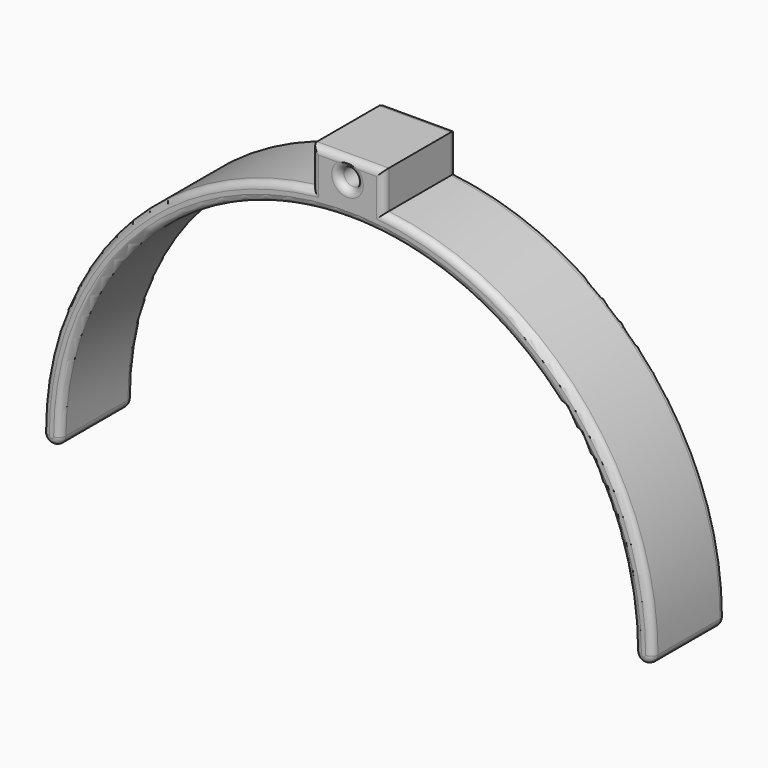
from build123d import *

# Parameters (mm, degrees)
F0_R         = 2.5
F1_DEPTH     = 25.4
F2_T1_DEPTH  = 29.525
F2_T4_ANGLE  = 180
F2_T6_ANGLE  = 180
F2_T8_ANGLE  = 180
F2_T12_ANGLE = 86.4550249792
F2_T17_DEPTH = 20.1152849193
F2_S18_R     = 85
F2_T19_DEPTH = 12
F2_T23_DEPTH = 20.1152849193
F2_S24_R     = 85
F2_T25_DEPTH = 12
F2_T29_ANGLE = 86.4550249792
F2_T37_ANGLE = 86.4550249792
F2_T41_DEPTH = 20.1152849193
F2_S42_R     = 85
F2_T43_DEPTH = 12
F2_T49_DEPTH = 20.1152849193
F2_S50_R     = 85
F2_T51_DEPTH = 12
F2_T54_ANGLE = 86.4550249792
F3_T3_ANGLE  = 180
F3_T6_ANGLE  = 180
F3_T9_ANGLE  = 180
F3_T12_ANGLE = 86.4550249792
F3_T16_DEPTH = 20.1152849193
F3_S17_R     = 85
F3_T18_DEPTH = 12
F3_T21_DEPTH = 29.525
F3_T24_DEPTH = 20.1152849193
F3_S25_R     = 85
F3_T26_DEPTH = 12
F3_T29_ANGLE = 86.4550249792
F3_T37_DEPTH = 20.1152849193
F3_S38_R     = 85
F3_T39_DEPTH = 12
F3_T42_ANGLE = 86.4550249792
F3_T48_ANGLE = 86.4550249792
F3_T52_DEPTH = 20.1152849193
F3_S53_R     = 85
F3_T54_DEPTH = 12


# Not quite as in the source:
# - a fillet or chamfer that OpenCascade refuses, or shapes differently, is made with other operations: its cross-section is extruded or revolved along the edge and cut away or added


with BuildPart() as f1:
    # F0 (on Front) → F1 (new body)
    with BuildSketch(Plane.XZ):
        with BuildLine():
            ThreePointArc((-80, 0), (0, 80), (80, 0))
            ThreePointArc((80, 0), (82.5, -2.5), (85, 0))
            ThreePointArc((85, 0), (63.5413251357, 56.4579489532), (10, 84.4097150807))
            Line((10, 84.4097150807), (10, 95))
            Line((10, 95), (0, 95))
            Line((0, 95), (-10, 95))
            Line((-10, 95), (-10, 84.4097150807))
            ThreePointArc((-10, 84.4097150807), (-63.5413251357, 56.4579489532), (-85, 0))
            ThreePointArc((-85, 0), (-82.5, -2.5), (-80, 0))
        make_face()
        with Locations((0, 89.7048575403)):
            Circle(F0_R, mode=Mode.SUBTRACT)
    extrude(amount=F1_DEPTH)

    # F2: fillet of radius 1.905 on 9 edges, made by hand

    # F2_s2 → F2_t1 (cut)
    with BuildSketch(Plane.YZ.offset(-14.7625)):
        with BuildLine():
            ThreePointArc((-25.4, 93.095), (-24.8420384182, 94.4420384182), (-23.495, 95))
            Line((-23.495, 95), (-25.4, 95))
            Line((-25.4, 95), (-25.4, 93.095))
        make_face()
    extrude(amount=F2_T1_DEPTH, mode=Mode.SUBTRACT)

    # F2_s3 → F2_t4 (revolve, cut)
    with BuildSketch(Plane.XY):
        with BuildLine():
            ThreePointArc((-85, -23.495), (-84.4420384182, -24.8420384182), (-83.095, -25.4))
            Line((-83.095, -25.4), (-85, -25.4))
            Line((-85, -25.4), (-85, -23.495))
        make_face()
    revolve(axis=Axis((-82.5, -25.4, 0), (0, -1, 0)), revolution_arc=F2_T4_ANGLE, mode=Mode.SUBTRACT)

    # F2_s5 → F2_t6 (revolve, cut)
    with BuildSketch(Plane.XY):
        with BuildLine():
            ThreePointArc((-81.905, -25.4), (-80.5579615818, -24.8420384182), (-80, -23.495))
            Line((-80, -23.495), (-80, -25.4))
            Line((-80, -25.4), (-81.905, -25.4))
        make_face()
    revolve(axis=Axis((0, -25.4, 0), (0, 1, 0)), revolution_arc=F2_T6_ANGLE, mode=Mode.SUBTRACT)

    # F2_s7 → F2_t8 (revolve, cut)
    with BuildSketch(Plane.XY):
        with BuildLine():
            ThreePointArc((81.905, -25.4), (80.5579615818, -24.8420384182), (80, -23.495))
            Line((80, -23.495), (80, -25.4))
            Line((80, -25.4), (81.905, -25.4))
        make_face()
    revolve(axis=Axis((82.5, -25.4, 0), (0, -1, 0)), revolution_arc=F2_T8_ANGLE, mode=Mode.SUBTRACT)


with BuildPart() as f2_tool10:
    # F2_s11 → F2_t12 (revolve)
    with BuildSketch(Plane.XY):
        with BuildLine():
            ThreePointArc((83.095, -25.4), (84.4420384182, -24.8420384182), (85, -23.495))
            Line((85, -23.495), (85, -25.4))
            Line((85, -25.4), (83.095, -25.4))
        make_face()
    revolve(axis=Axis((0, -25.4, 0), (0, -1, 0)), revolution_arc=F2_T12_ANGLE)

    split(bisect_by=Plane.YZ.offset(10), keep=Keep.TOP)


with BuildPart() as f1_1:
    add(f1.part)

    # F2_t9: cut F2_tool10
    add(f2_tool10.part, mode=Mode.SUBTRACT)


with BuildPart() as f2_tool15:
    # F2_s16 → F2_t17 (new body)
    with BuildSketch(Plane.XY.offset(79.6472150807)):
        with BuildLine():
            ThreePointArc((8.095, -25.4), (9.4420384182, -24.8420384182), (10, -23.495))
            Line((10, -23.495), (10, -25.4))
            Line((10, -25.4), (8.095, -25.4))
        make_face()
    extrude(amount=F2_T17_DEPTH)

    # F2_s18 → F2_t19 (cut, symmetric)
    with BuildSketch(Plane.XZ.offset(24.4)):
        Circle(F2_S18_R)
    extrude(amount=F2_T19_DEPTH, both=True, mode=Mode.SUBTRACT)


with BuildPart() as f1_2:
    add(f1_1.part)

    # F2_t14: cut F2_tool15
    add(f2_tool15.part, mode=Mode.SUBTRACT)


with BuildPart() as f2_tool21:
    # F2_s22 → F2_t23 (new body)
    with BuildSketch(Plane.XY.offset(99.7625)):
        with BuildLine():
            ThreePointArc((-8.095, -25.4), (-9.4420384182, -24.8420384182), (-10, -23.495))
            Line((-10, -23.495), (-10, -25.4))
            Line((-10, -25.4), (-8.095, -25.4))
        make_face()
    extrude(amount=-F2_T23_DEPTH)

    # F2_s24 → F2_t25 (cut, symmetric)
    with BuildSketch(Plane.XZ.offset(24.4)):
        Circle(F2_S24_R)
    extrude(amount=F2_T25_DEPTH, both=True, mode=Mode.SUBTRACT)


with BuildPart() as f1_3:
    add(f1_2.part)

    # F2_t20: cut F2_tool21
    add(f2_tool21.part, mode=Mode.SUBTRACT)


with BuildPart() as f2_tool27:
    # F2_s28 → F2_t29 (revolve)
    with BuildSketch(Plane(origin=(0, 0, 0), x_dir=(0, 1, 0), z_dir=(0.9980865701, 0, 0.0618320187))):
        with BuildLine():
            ThreePointArc((-25.4, 83.095), (-24.8420384182, 84.4420384182), (-23.495, 85))
            Line((-23.495, 85), (-25.4, 85))
            Line((-25.4, 85), (-25.4, 83.095))
        make_face()
    revolve(axis=Axis((0, -25.4, 0), (0, -1, 0)), revolution_arc=F2_T29_ANGLE)

    split(bisect_by=Plane.YZ.offset(-10), keep=Keep.BOTTOM)


with BuildPart() as f1_4:
    add(f1_3.part)

    # F2_t26: cut F2_tool27
    add(f2_tool27.part, mode=Mode.SUBTRACT)

    # F2_s31 → F2_t32 (revolve, cut)
    with BuildSketch(Plane.XY.offset(89.7048575403)):
        with BuildLine():
            ThreePointArc((4.405, -25.4), (3.0579615818, -24.8420384182), (2.5, -23.495))
            Line((2.5, -23.495), (2.5, -25.4))
            Line((2.5, -25.4), (4.405, -25.4))
        make_face()
    revolve(axis=Axis((0, -25.4, 89.7048575403), (0, -1, 0)), mode=Mode.SUBTRACT)


with BuildPart() as f2_tool35:
    # F2_s36 → F2_t37 (revolve)
    with BuildSketch(Plane.XY):
        with BuildLine():
            ThreePointArc((83.095, -25.4), (84.4420384182, -24.8420384182), (85, -23.495))
            Line((85, -23.495), (85, -25.4))
            Line((85, -25.4), (83.095, -25.4))
        make_face()
    revolve(axis=Axis((0, -25.4, 0), (0, -1, 0)), revolution_arc=F2_T37_ANGLE)

    split(bisect_by=Plane.YZ.offset(10), keep=Keep.BOTTOM)


with BuildPart() as f2_tool39:
    # F2_s40 → F2_t41 (new body)
    with BuildSketch(Plane.XY.offset(79.6472150807)):
        with BuildLine():
            ThreePointArc((8.095, -25.4), (9.4420384182, -24.8420384182), (10, -23.495))
            Line((10, -23.495), (10, -25.4))
            Line((10, -25.4), (8.095, -25.4))
        make_face()
    extrude(amount=F2_T41_DEPTH)

    # F2_s42 → F2_t43 (intersect, symmetric)
    with BuildSketch(Plane.XZ.offset(24.4)):
        Circle(F2_S42_R)
    extrude(amount=F2_T43_DEPTH, both=True, mode=Mode.INTERSECT)


with BuildPart() as f2_tool35_1:
    add(f2_tool35.part)

    # F2_t44: intersect F2_tool39
    add(f2_tool39.part, mode=Mode.INTERSECT)


with BuildPart() as f1_5:
    add(f1_4.part)

    # F2_t33: cut F2_tool35
    add(f2_tool35_1.part, mode=Mode.SUBTRACT)


with BuildPart() as f2_tool47:
    # F2_s48 → F2_t49 (new body)
    with BuildSketch(Plane.XY.offset(99.7625)):
        with BuildLine():
            ThreePointArc((-8.095, -25.4), (-9.4420384182, -24.8420384182), (-10, -23.495))
            Line((-10, -23.495), (-10, -25.4))
            Line((-10, -25.4), (-8.095, -25.4))
        make_face()
    extrude(amount=-F2_T49_DEPTH)

    # F2_s50 → F2_t51 (intersect, symmetric)
    with BuildSketch(Plane.XZ.offset(24.4)):
        Circle(F2_S50_R)
    extrude(amount=F2_T51_DEPTH, both=True, mode=Mode.INTERSECT)


with BuildPart() as f2_tool52:
    # F2_s53 → F2_t54 (revolve)
    with BuildSketch(Plane(origin=(0, 0, 0), x_dir=(0, 1, 0), z_dir=(0.9980865701, 0, 0.0618320187))):
        with BuildLine():
            ThreePointArc((-25.4, 83.095), (-24.8420384182, 84.4420384182), (-23.495, 85))
            Line((-23.495, 85), (-25.4, 85))
            Line((-25.4, 85), (-25.4, 83.095))
        make_face()
    revolve(axis=Axis((0, -25.4, 0), (0, -1, 0)), revolution_arc=F2_T54_ANGLE)

    split(bisect_by=Plane.YZ.offset(-10), keep=Keep.TOP)


with BuildPart() as f2_tool47_1:
    add(f2_tool47.part)

    # F2_t56: intersect F2_tool52
    add(f2_tool52.part, mode=Mode.INTERSECT)


with BuildPart() as f1_6:
    add(f1_5.part)

    # F2_t45: cut F2_tool47
    add(f2_tool47_1.part, mode=Mode.SUBTRACT)

    # F3: fillet of radius 1.905 on 9 edges, made by hand


with BuildPart() as f3_tool1:
    # F3_s2 → F3_t3 (revolve)
    with BuildSketch(Plane.XY):
        with BuildLine():
            ThreePointArc((-85, -1.905), (-84.4420384182, -0.5579615818), (-83.095, 0))
            Line((-83.095, 0), (-85, 0))
            Line((-85, 0), (-85, -1.905))
        make_face()
    revolve(axis=Axis((-82.5, 0, 0), (0, -1, 0)), revolution_arc=F3_T3_ANGLE)


with BuildPart() as f3_tool4:
    # F3_s5 → F3_t6 (revolve)
    with BuildSketch(Plane.XY):
        with BuildLine():
            ThreePointArc((-80, -1.905), (-80.5579615818, -0.5579615818), (-81.905, 0))
            Line((-81.905, 0), (-80, 0))
            Line((-80, 0), (-80, -1.905))
        make_face()
    revolve(axis=Axis((0, 0, 0), (0, 1, 0)), revolution_arc=F3_T6_ANGLE)


with BuildPart() as f3_tool7:
    # F3_s8 → F3_t9 (revolve)
    with BuildSketch(Plane.XY):
        with BuildLine():
            ThreePointArc((80, -1.905), (80.5579615818, -0.5579615818), (81.905, 0))
            Line((81.905, 0), (80, 0))
            Line((80, 0), (80, -1.905))
        make_face()
    revolve(axis=Axis((82.5, 0, 0), (0, -1, 0)), revolution_arc=F3_T9_ANGLE)


with BuildPart() as f3_tool10:
    # F3_s11 → F3_t12 (revolve)
    with BuildSketch(Plane.XY):
        with BuildLine():
            ThreePointArc((85, -1.905), (84.4420384182, -0.5579615818), (83.095, 0))
            Line((83.095, 0), (85, 0))
            Line((85, 0), (85, -1.905))
        make_face()
    revolve(axis=Axis((0, 0, 0), (0, -1, 0)), revolution_arc=F3_T12_ANGLE)

    split(bisect_by=Plane.YZ.offset(10), keep=Keep.TOP)


with BuildPart() as f3_tool14:
    # F3_s15 → F3_t16 (new body)
    with BuildSketch(Plane.XY.offset(79.6472150807)):
        with BuildLine():
            ThreePointArc((10, -1.905), (9.4420384182, -0.5579615818), (8.095, 0))
            Line((8.095, 0), (10, 0))
            Line((10, 0), (10, -1.905))
        make_face()
    extrude(amount=F3_T16_DEPTH)

    # F3_s17 → F3_t18 (cut, symmetric)
    with BuildSketch(Plane.XZ.offset(1)):
        Circle(F3_S17_R)
    extrude(amount=F3_T18_DEPTH, both=True, mode=Mode.SUBTRACT)


with BuildPart() as f3_tool19:
    # F3_s20 → F3_t21 (new body)
    with BuildSketch(Plane.YZ.offset(14.7625)):
        with BuildLine():
            ThreePointArc((-1.905, 95), (-0.5579615818, 94.4420384182), (0, 93.095))
            Line((0, 93.095), (0, 95))
            Line((0, 95), (-1.905, 95))
        make_face()
    extrude(amount=-F3_T21_DEPTH)


with BuildPart() as f3_tool22:
    # F3_s23 → F3_t24 (new body)
    with BuildSketch(Plane.XY.offset(99.7625)):
        with BuildLine():
            ThreePointArc((-10, -1.905), (-9.4420384182, -0.5579615818), (-8.095, 0))
            Line((-8.095, 0), (-10, 0))
            Line((-10, 0), (-10, -1.905))
        make_face()
    extrude(amount=-F3_T24_DEPTH)

    # F3_s25 → F3_t26 (cut, symmetric)
    with BuildSketch(Plane.XZ.offset(1)):
        Circle(F3_S25_R)
    extrude(amount=F3_T26_DEPTH, both=True, mode=Mode.SUBTRACT)


with BuildPart() as f3_tool27:
    # F3_s28 → F3_t29 (revolve)
    with BuildSketch(Plane(origin=(0, 0, 0), x_dir=(0, 1, 0), z_dir=(0.9980865701, 0, 0.0618320187))):
        with BuildLine():
            ThreePointArc((-1.905, 85), (-0.5579615818, 84.4420384182), (0, 83.095))
            Line((0, 83.095), (0, 85))
            Line((0, 85), (-1.905, 85))
        make_face()
    revolve(axis=Axis((0, 0, 0), (0, -1, 0)), revolution_arc=F3_T29_ANGLE)

    split(bisect_by=Plane.YZ.offset(-10), keep=Keep.BOTTOM)


with BuildPart() as f3_tool31:
    # F3_s32 → F3_t33 (revolve)
    with BuildSketch(Plane.XY.offset(89.7048575403)):
        with BuildLine():
            ThreePointArc((2.5, -1.905), (3.0579615818, -0.5579615818), (4.405, 0))
            Line((4.405, 0), (2.5, 0))
            Line((2.5, 0), (2.5, -1.905))
        make_face()
    revolve(axis=Axis((0, 0, 89.7048575403), (0, -1, 0)))


with BuildPart() as f3_tool35:
    # F3_s36 → F3_t37 (new body)
    with BuildSketch(Plane.XY.offset(79.6472150807)):
        with BuildLine():
            ThreePointArc((10, -1.905), (9.4420384182, -0.5579615818), (8.095, 0))
            Line((8.095, 0), (10, 0))
            Line((10, 0), (10, -1.905))
        make_face()
    extrude(amount=F3_T37_DEPTH)

    # F3_s38 → F3_t39 (intersect, symmetric)
    with BuildSketch(Plane.XZ.offset(1)):
        Circle(F3_S38_R)
    extrude(amount=F3_T39_DEPTH, both=True, mode=Mode.INTERSECT)


with BuildPart() as f3_tool40:
    # F3_s41 → F3_t42 (revolve)
    with BuildSketch(Plane.XY):
        with BuildLine():
            ThreePointArc((85, -1.905), (84.4420384182, -0.5579615818), (83.095, 0))
            Line((83.095, 0), (85, 0))
            Line((85, 0), (85, -1.905))
        make_face()
    revolve(axis=Axis((0, 0, 0), (0, -1, 0)), revolution_arc=F3_T42_ANGLE)

    split(bisect_by=Plane.YZ.offset(10), keep=Keep.BOTTOM)


with BuildPart() as f3_tool35_1:
    add(f3_tool35.part)

    # F3_t44: intersect F3_tool40
    add(f3_tool40.part, mode=Mode.INTERSECT)


with BuildPart() as f3_tool46:
    # F3_s47 → F3_t48 (revolve)
    with BuildSketch(Plane(origin=(0, 0, 0), x_dir=(0, 1, 0), z_dir=(0.9980865701, 0, 0.0618320187))):
        with BuildLine():
            ThreePointArc((-1.905, 85), (-0.5579615818, 84.4420384182), (0, 83.095))
            Line((0, 83.095), (0, 85))
            Line((0, 85), (-1.905, 85))
        make_face()
    revolve(axis=Axis((0, 0, 0), (0, -1, 0)), revolution_arc=F3_T48_ANGLE)

    split(bisect_by=Plane.YZ.offset(-10), keep=Keep.TOP)


with BuildPart() as f3_tool50:
    # F3_s51 → F3_t52 (new body)
    with BuildSketch(Plane.XY.offset(99.7625)):
        with BuildLine():
            ThreePointArc((-10, -1.905), (-9.4420384182, -0.5579615818), (-8.095, 0))
            Line((-8.095, 0), (-10, 0))
            Line((-10, 0), (-10, -1.905))
        make_face()
    extrude(amount=-F3_T52_DEPTH)

    # F3_s53 → F3_t54 (intersect, symmetric)
    with BuildSketch(Plane.XZ.offset(1)):
        Circle(F3_S53_R)
    extrude(amount=F3_T54_DEPTH, both=True, mode=Mode.INTERSECT)


with BuildPart() as f3_tool46_1:
    add(f3_tool46.part)

    # F3_t55: intersect F3_tool50
    add(f3_tool50.part, mode=Mode.INTERSECT)


with BuildPart() as f1_7:
    add(f1_6.part)

    # F3_t56: cut F3_tool1, F3_tool4, F3_tool7, F3_tool10, F3_tool14, F3_tool19, F3_tool22, F3_tool27, F3_tool31, F3_tool35, F3_tool46
    add([f3_tool1.part, f3_tool4.part, f3_tool7.part, f3_tool10.part, f3_tool14.part, f3_tool19.part, f3_tool22.part, f3_tool27.part, f3_tool31.part, f3_tool35_1.part, f3_tool46_1.part], mode=Mode.SUBTRACT)


solid = f1_7.part
